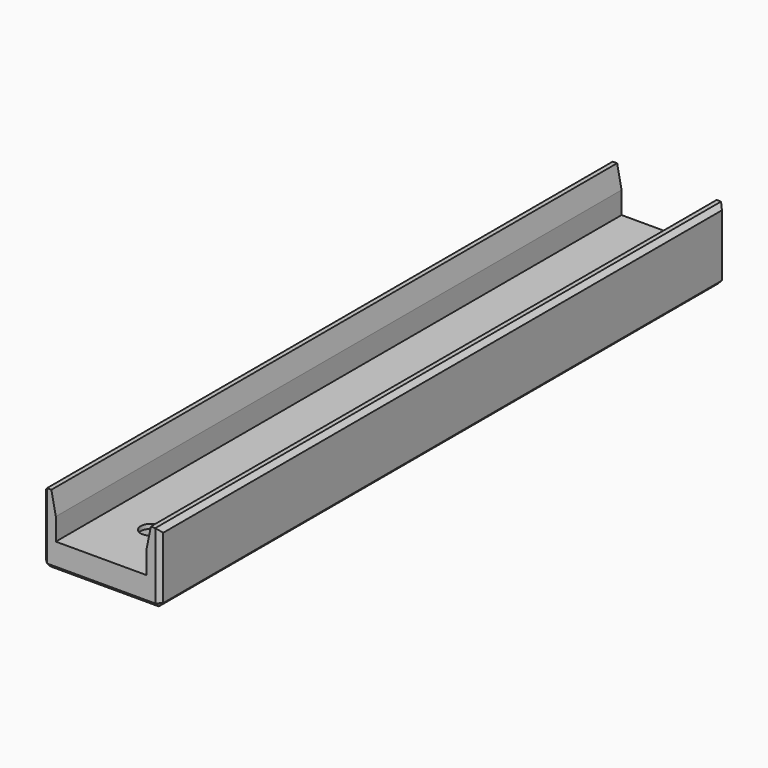
from build123d import *

# Parameters (mm, degrees)
F1_DEPTH  = 160
F2_R      = 2.25
F3_DEPTH  = 16.001
F4_SIZE2  = 1
F4_SIZE   = 5
F5_SIZE2  = 5
F5_SIZE   = 1
F7_DEPTH  = 5
F8_R      = 2.25
F9_DEPTH  = 2
F10_SIZE  = 1.5
F11_SIZE  = 1
F12_W     = 12
F12_H     = 6
F12_W_2   = 4
F12_H_2   = 14
F13_DEPTH = 1


# Not quite as in the source:
# - a feature names something its author has since deleted; it is built from what else it names


with BuildPart() as f1:
    # F0 (on Front) → F1 (new body)
    with BuildSketch(Plane.XZ):
        Polygon((0, 16), (0, 0), (26.5, 0), (26.5, 16), (23.5, 16), (23.5, 6), (3, 6), (3, 16), align=None)
    extrude(amount=F1_DEPTH)

    # F2 (on face) → F3 (cut, through all)
    with BuildSketch(Plane(origin=(0, 0, 0), x_dir=(1, 0, 0), z_dir=(0, 0, -1))):
        with Locations((13.25, 146)):
            Circle(F2_R)
    extrude(amount=-F3_DEPTH, mode=Mode.SUBTRACT)

    # F4
    f4_edges = [f1.edges().sort_by_distance(p)[0] for p in [
        (23.5, -80, 16),
    ]]
    f4_side = f1.faces().sort_by_distance((23.5, -80, 11))[0]
    chamfer(f4_edges, length=F4_SIZE, length2=F4_SIZE2, reference=f4_side)

    # F5
    f5_edges = [f1.edges().sort_by_distance(p)[0] for p in [
        (3, -80, 16),
    ]]
    f5_side = f1.faces().sort_by_distance((1.5, -80, 16))[0]
    chamfer(f5_edges, length=F5_SIZE, length2=F5_SIZE2, reference=f5_side)

    # F6 (on face) → F7 (cut)
    with BuildSketch(Plane(origin=(0, 0, 0), x_dir=(1, 0, 0), z_dir=(0, 0, -1))):
        Polygon((15.2707259422, 149.5), (11.2292740578, 149.5), (9.2085481157, 146), (11.2292740578, 142.5), (15.2707259422, 142.5), (17.2914518843, 146), align=None)
    extrude(amount=-F7_DEPTH, mode=Mode.SUBTRACT)

    # F8 (on face) → F9 (join)
    with BuildSketch(Plane(origin=(0, 0, 0), x_dir=(1, 0, 0), z_dir=(0, 0, -1))):
        Polygon((15.2707259422, 149.5), (11.2292740578, 149.5), (9.2085481157, 146), (11.2292740578, 142.5), (15.2707259422, 142.5), (17.2914518843, 146), align=None)
        with Locations((13.25, 146)):
            Circle(F8_R, mode=Mode.SUBTRACT)
    extrude(amount=-F9_DEPTH)

    # F10
    f10_edges = [f1.edges().sort_by_distance(p)[0] for p in [
        (11, -146, 0),
    ]]
    chamfer(f10_edges, length=F10_SIZE)

    # F11
    f11_edges = [f1.edges().sort_by_distance(p)[0] for p in [
        (0, -80, 0),
        (13.25, 0, 0),
        (26.5, -80, 0),
        (13.25, -160, 0),
        (0, 0, 8),
        (26.5, 0, 8),
        (0, -160, 8),
        (26.5, -160, 8),
        (26.5, -80, 16),
        (0, -80, 16),
    ]]
    chamfer(f11_edges, length=F11_SIZE)

    # F12 (on face) → F13 (cut)
    with BuildSketch(Plane(origin=(0, 0, 0), x_dir=(1, 0, 0), z_dir=(0, 0, -1))):
        Polygon((6.25, 18), (6.25, 10), (20.25, 10), (20.25, 18), (20.25, 32), (20.25, 33), (20.25, 40), (6.25, 40), (6.25, 33), align=None)
        with Locations((13.25, 14)):
            Rectangle(F12_W, F12_H, mode=Mode.SUBTRACT)
        with Locations((9.25, 25)):
            Rectangle(F12_W_2, F12_H_2, mode=Mode.SUBTRACT)
        Polygon((15.7156598493, 18), (12.25, 18), (12.25, 32), (19.25, 32), (19.25, 18), (16.2156598493, 18), (17.4656598493, 21), (16.4656598493, 21), (16.4656598493, 26), (15.4656598493, 26), (15.4656598493, 21), (14.4656598493, 21), align=None, mode=Mode.SUBTRACT)
        with Locations((13.25, 36)):
            Rectangle(F12_W, F12_H, mode=Mode.SUBTRACT)
    extrude(amount=-F13_DEPTH, mode=Mode.SUBTRACT)


solid = f1.part
